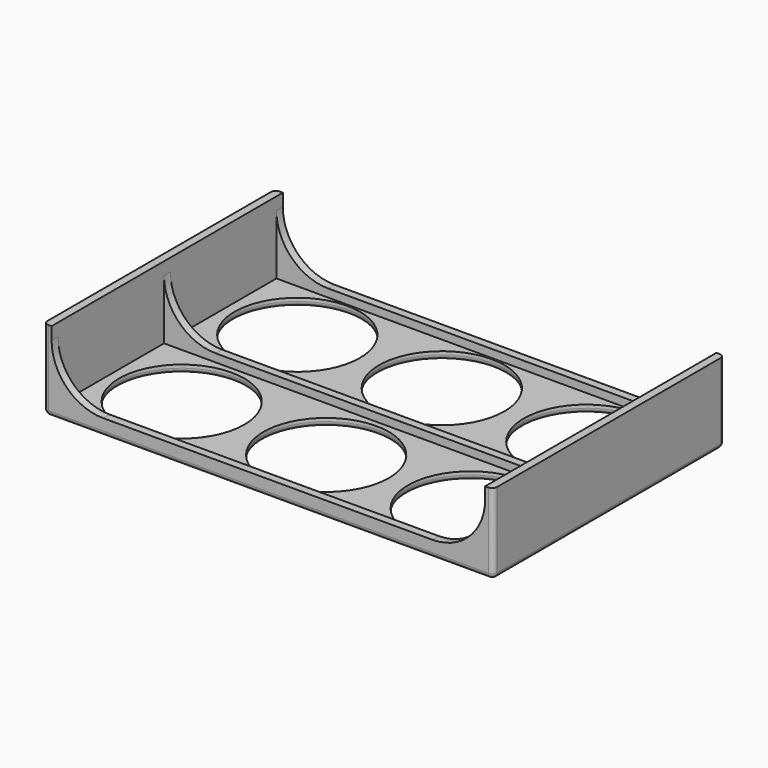
from build123d import *

# Parameters (mm, degrees)
F0_W     = 140
F0_H     = 90
F1_DEPTH = 25
F2_T     = -2.5
F4_W     = 140
F4_H     = 90
F4_R     = 19.5
F5_DEPTH = 25
F6_R     = 1.49999
F7_W     = 135
F7_H     = 2.5
F8_DEPTH = 22.5
F9_DEPTH = 90.001


# Not quite as in the source:
# - a fillet or chamfer is up to 0.001 mm smaller than in the source, because OpenCascade refuses the exact size


with BuildPart() as f1:
    # F0 (on Top) → F1 (new body)
    with BuildSketch(Plane.XY):
        with Locations((-70, 0)):
            Rectangle(F0_W, F0_H)
    extrude(amount=F1_DEPTH)

    # F2
    f2_openings = [f1.faces().sort_by_distance(p)[0] for p in [
        (-70, 0, 25),
    ]]
    offset(amount=F2_T, openings=f2_openings)

    # F4 (on face) → F5 (intersect)
    with BuildSketch(Plane(origin=(0, 0, 0), x_dir=(1, 0, 0), z_dir=(0, 0, -1))):
        with Locations((-70, 0)):
            Rectangle(F4_W, F4_H)
        with Locations((-115, -22.5)):
            Circle(F4_R, mode=Mode.SUBTRACT)
        with Locations((-70, -22.5)):
            Circle(F4_R, mode=Mode.SUBTRACT)
        with Locations((-25, -22.5)):
            Circle(F4_R, mode=Mode.SUBTRACT)
        with Locations((-115, 22.5)):
            Circle(F4_R, mode=Mode.SUBTRACT)
        with Locations((-70, 22.5)):
            Circle(F4_R, mode=Mode.SUBTRACT)
        with Locations((-25, 22.5)):
            Circle(F4_R, mode=Mode.SUBTRACT)
    extrude(amount=-F5_DEPTH, mode=Mode.INTERSECT)

    # F6 (radius 1.5 in the source; OpenCascade refuses exactly that, so slightly less here)
    f6_edges = [f1.edges().sort_by_distance(p)[0] for p in [
        (-70, -45, 0),
        (-140, 0, 0),
        (-70, 45, 0),
        (0, 0, 0),
        (-134.5, 22.5, 0),
        (-89.5, 22.5, 0),
        (-44.5, 22.5, 0),
        (-134.5, -22.5, 0),
        (-89.5, -22.5, 0),
        (-44.5, -22.5, 0),
        (-140, 45, 12.5),
        (-140, -45, 12.5),
        (0, -45, 12.5),
        (0, 45, 12.5),
    ]]
    fillet(f6_edges, radius=F6_R)

    # F7 (on face) → F8 (join)
    with BuildSketch(Plane.XY.offset(2.5)):
        with Locations((-70, 0)):
            Rectangle(F7_W, F7_H)
    extrude(amount=F8_DEPTH)

    # F3 (on face) → F9 (cut, through all)
    with BuildSketch(Plane.XZ.offset(45)):
        with BuildLine():
            Line((-2.5, 25), (-137.5, 25))
            Line((-137.5, 25), (-137.5, 21.0707051933))
            ThreePointArc((-137.5, 21.0707051933), (-132.7929994273, 9.7070005727), (-121.4292948067, 5))
            Line((-121.4292948067, 5), (-18.9261284359, 5))
            ThreePointArc((-18.9261284359, 5), (-7.3111016302, 9.8111016302), (-2.5, 21.4261284359))
            Line((-2.5, 21.4261284359), (-2.5, 25))
        make_face()
    extrude(amount=-F9_DEPTH, mode=Mode.SUBTRACT)


solid = f1.part
